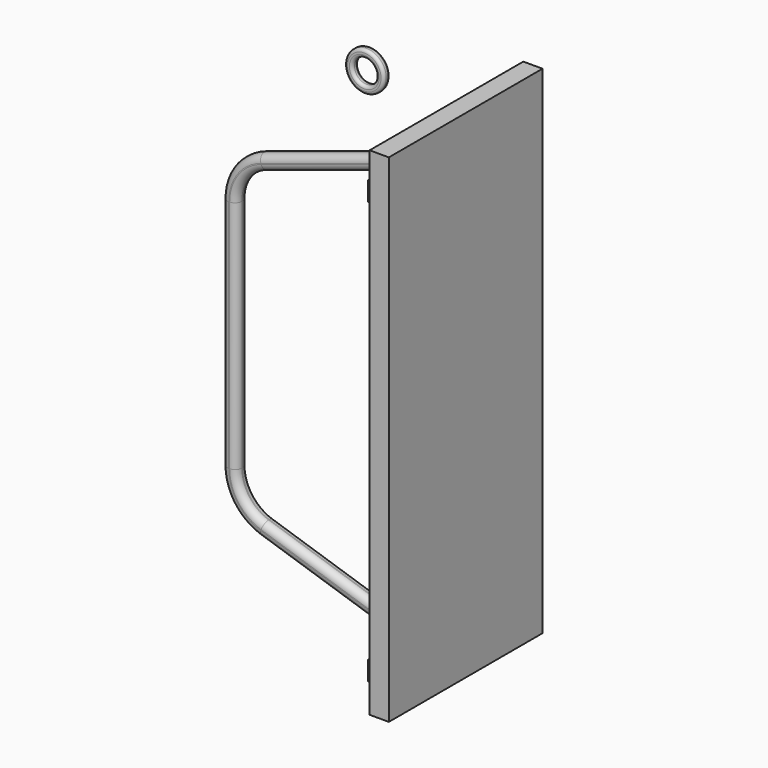
from build123d import *

# Parameters (mm, degrees)
F1_DEPTH = 75
F2_DEPTH = 15
F3_R     = 7
F4_R     = 20.4711735864
F4_R_2   = 12.4711735864
F5_DEPTH = 8
F6_R     = 3
F4_W     = 20
F4_H     = 517.5366248004
F7_DEPTH = 100


# Not quite as in the source:
# - a feature names something its author has since deleted; it is built from what else it names


with BuildPart() as f1:
    # F0 (on Front) → F1 (new body, symmetric)
    with BuildSketch(Plane.XZ):
        Polygon((6.3377187523, 17.2496383322), (-13.9010772109, 17.2386454604), (-13.9010772109, 15.8079492705), (-13.9010772109, 0.0360159069), (-13.9010772109, -2.7503587176), (6.3485819185, -2.7503587176), align=None)
    extrude(amount=F1_DEPTH, both=True)


with BuildPart() as f1b:
    # F0 (on Front) → F1, piece 2 (new body, symmetric)
    with BuildSketch(Plane.XZ):
        Polygon((6.1097859569, 436.8929690868), (6.0989227891, 456.8929690868), (-13.9010772109, 456.8929690868), (-13.9010772109, 455.1017939944), (-13.9010772109, 439.3298606308), (-13.9010772109, 436.8821000186), align=None)
    extrude(amount=F1_DEPTH, both=True)


with BuildPart() as f2:
    # F0 (on Front) → F2 (new body)
    with BuildSketch(Plane.XZ):
        with BuildLine():
            Line((-13.9010772109, 439.3298606308), (-13.9010772109, 455.1017939944))
            Line((-13.9010772109, 455.1017939944), (-175.5806849811, 402.5689049507))
            ThreePointArc((-175.5806849811, 402.5689049507), (-203.309581291, 382.4226825268), (-213.9010772109, 349.8254099002))
            Line((-213.9010772109, 349.8254099002), (-213.9010772109, 105.3124000012))
            ThreePointArc((-213.9010772109, 105.3124000012), (-203.309581291, 72.7151273745), (-175.5806849811, 52.5689049507))
            Line((-175.5806849811, 52.5689049507), (-13.9010772109, 0.0360159069))
            Line((-13.9010772109, 0.0360159069), (-13.9010772109, 15.8079492705))
            Line((-13.9010772109, 15.8079492705), (-170.9454300655, 66.8347526951))
            ThreePointArc((-170.9454300655, 66.8347526951), (-191.1743263754, 81.5319061589), (-198.9010772109, 105.3124000012))
            Line((-198.9010772109, 105.3124000012), (-198.9010772109, 349.8254099002))
            ThreePointArc((-198.9010772109, 349.8254099002), (-191.1743263754, 373.6059037424), (-170.9454300655, 388.3030572062))
            Line((-170.9454300655, 388.3030572062), (-13.9010772109, 439.3298606308))
        make_face()
    extrude(amount=F2_DEPTH)

    # F3
    f3_edges = [f2.edges().sort_by_distance(p)[0] for p in [
        (-94.740881, -15, 428.835349),
        (-94.740881, 0, 428.835349),
        (-92.423254, -15, 413.816459),
        (-92.423254, 0, 413.816459),
    ]]
    fillet(f3_edges, radius=F3_R)


with BuildPart() as f5:
    # F4 (on Front) → F5 (new body)
    with BuildSketch(Plane.XZ):
        with Locations((-71.3653936982, 509.9469423294)):
            Circle(F4_R)
        with Locations((-71.3653936982, 509.9469423294)):
            Circle(F4_R_2, mode=Mode.SUBTRACT)
    extrude(amount=F5_DEPTH)

    # F6
    f6_edges = [f5.edges().sort_by_distance(p)[0] for p in [
        (-91.836567, -8, 509.946942),
        (-91.836567, 0, 509.946942),
        (-83.836567, 0, 509.946942),
        (-83.836567, -8, 509.946942),
    ]]
    fillet(f6_edges, radius=F6_R)


with BuildPart() as f7:
    # F4 (on Front) → F7 (new body, symmetric)
    with BuildSketch(Plane.XZ):
        with Locations((17.8187572956, 242.5810175482)):
            Rectangle(F4_W, F4_H)
    extrude(amount=F7_DEPTH, both=True)


solid = Compound([f1.part, f1b.part, f2.part, f5.part, f7.part])
